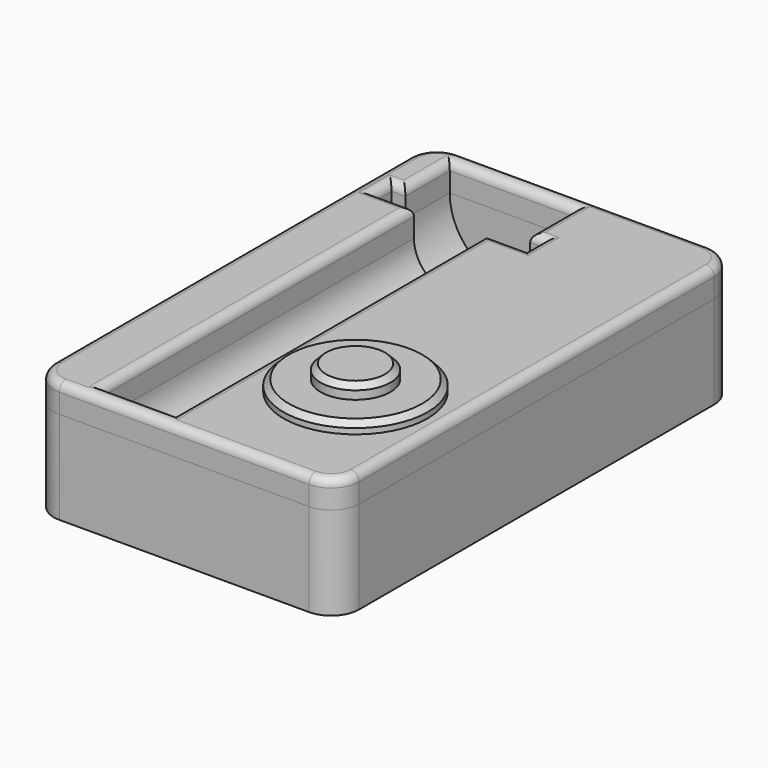
from build123d import *

# Parameters (mm, degrees)
F0_W           = 55
F0_H           = 90
F1_DEPTH       = 16.75
F4_R           = 13
F5_DEPTH       = 2
F7_W           = 55
F7_H           = 90
F8_DEPTH       = 5
F9_R           = 13
F10_DEPTH      = 2
F11_R          = 6.3
F12_DEPTH      = 23.751
F13_R          = 5
F13_2_R        = 5
F14_SIZE       = 1
F15_T1_DEPTH   = 22.5
F15_T3_DEPTH   = 13.75
F15_T5_DEPTH   = 6.25
F15_T7_DEPTH   = 4
F15_T9_DEPTH   = 11
F15_T11_DEPTH  = 73.75
F15_T13_DEPTH  = 13
F15_T15_DEPTH  = 11
F15_T17_DEPTH  = 6.25
F15_T19_DEPTH  = 80
F15_T21_DEPTH  = 45
F15_T24_ANGLE  = 90
F15_T26_ANGLE  = 90
F15_T28_ANGLE  = 90
F15_T30_ANGLE  = 90
F15_T35_DEPTH  = 26.25
F15_T39_DEPTH  = 17.5
F15_T46_DEPTH  = 26.25
F15_T50_DEPTH  = 17.5
F15_T57_DEPTH  = 10
F15_T61_DEPTH  = 7.75
F15_T68_DEPTH  = 7.75
F15_T72_DEPTH  = 14.75
F15_T79_DEPTH  = 77.5
F15_T83_DEPTH  = 16.75
F15_T90_DEPTH  = 77.5
F15_T94_DEPTH  = 16.75
F15_T101_DEPTH = 7.75
F15_T105_DEPTH = 14.75
F15_T112_DEPTH = 10
F15_T116_DEPTH = 7.75
F16_R          = 6.3
F17_DEPTH      = 26.25
F18_SIZE       = 1


# Not quite as in the source:
# - a fillet or chamfer that OpenCascade refuses, or shapes differently, is made with other operations: its cross-section is extruded or revolved along the edge and cut away or added


with BuildPart() as f1:
    # F0 (on Top) → F1 (new body)
    with BuildSketch(Plane.XY):
        Rectangle(F0_W, F0_H)
    extrude(amount=-F1_DEPTH)

    # F2 (on face) → F3 (revolve, cut)
    with BuildSketch(Plane.XY):
        Polygon((0.75, 42), (-10.5, 42), (-10.5, -42), (-4, -42), (-4, 28), (3.25, 28), (3.25, 32), (0.75, 32), align=None)
    revolve(axis=Axis((-10.5, 0, 0), (0, 1, 0)), mode=Mode.SUBTRACT)


with BuildPart() as f5:
    # F4 (on face) → F5 (new body)
    with BuildSketch(Plane.XY):
        with Locations((12.5, -25)):
            Circle(F4_R)
    extrude(amount=F5_DEPTH)


with BuildPart() as f8:
    # F7 (on face) → F8 (new body)
    with BuildSketch(Plane.XY):
        Rectangle(F7_W, F7_H)
        Polygon((-21.75, 42), (0.75, 42), (0.75, 32), (3.25, 32), (3.25, 28), (-4, 28), (-4, -42), (-17, -42), (-17, 28), (-24.25, 28), (-24.25, 32), (-21.75, 32), align=None, mode=Mode.SUBTRACT)
    extrude(amount=F8_DEPTH)


with BuildPart() as f10:
    # F9 (on face) → F10 (new body)
    with BuildSketch(Plane.XY.offset(5)):
        with Locations((11.75, -21.1021695286)):
            Circle(F9_R)
    extrude(amount=F10_DEPTH)


with BuildPart() as f12_tool:
    # F11 (on face) → F12 (new body, through all)
    with BuildSketch(Plane.XY.offset(7)):
        with Locations((11.75, -21.1021695286)):
            Circle(F11_R)
    extrude(amount=-F12_DEPTH)


with BuildPart() as f1_1:
    add(f1.part)

    # F12: cut by f12_tool
    add(f12_tool.part, mode=Mode.SUBTRACT)

    # F13
    f13_edges = [f1_1.edges().sort_by_distance(p)[0] for p in [
        (-27.5, -45, -8.375),
        (27.5, -45, -8.375),
        (27.5, 45, -8.375),
        (-27.5, 45, -8.375),
    ]]
    fillet(f13_edges, radius=F13_R)


with BuildPart() as f8_1:
    add(f8.part)

    # F12: cut by f12_tool
    add(f12_tool.part, mode=Mode.SUBTRACT)

    # F13#2
    f13_2_edges = [f8_1.edges().sort_by_distance(p)[0] for p in [
        (-27.5, -45, 2.5),
        (27.5, -45, 2.5),
        (27.5, 45, 2.5),
        (-27.5, 45, 2.5),
    ]]
    fillet(f13_2_edges, radius=F13_2_R)

    # F15: fillet of radius 1.5 on 13 edges, made by hand

    # F15_s2 → F15_t1 (cut)
    with BuildSketch(Plane.YZ.offset(-21.75)):
        with BuildLine():
            ThreePointArc((43.5, 5), (42.4393398282, 4.5606601718), (42, 3.5))
            Line((42, 3.5), (42, 5))
            Line((42, 5), (43.5, 5))
        make_face()
    extrude(amount=F15_T1_DEPTH, mode=Mode.SUBTRACT)

    # F15_s4 → F15_t3 (cut)
    with BuildSketch(Plane.XZ.offset(-42)):
        with BuildLine():
            ThreePointArc((-23.25, 5), (-22.1893398282, 4.5606601718), (-21.75, 3.5))
            Line((-21.75, 3.5), (-21.75, 5))
            Line((-21.75, 5), (-23.25, 5))
        make_face()
        with BuildLine():
            ThreePointArc((2.25, 5), (1.1893398282, 4.5606601718), (0.75, 3.5))
            Line((0.75, 3.5), (0.75, 5))
            Line((0.75, 5), (2.25, 5))
        make_face()
    extrude(amount=F15_T3_DEPTH, mode=Mode.SUBTRACT)

    # F15_s6 → F15_t5 (cut)
    with BuildSketch(Plane.YZ.offset(-24.25)):
        with BuildLine():
            ThreePointArc((33.5, 5), (32.4393398282, 4.5606601718), (32, 3.5))
            Line((32, 3.5), (32, 5))
            Line((32, 5), (33.5, 5))
        make_face()
    extrude(amount=F15_T5_DEPTH, mode=Mode.SUBTRACT)

    # F15_s8 → F15_t7 (cut)
    with BuildSketch(Plane.XZ.offset(-32)):
        with BuildLine():
            ThreePointArc((-25.75, 5), (-24.6893398282, 4.5606601718), (-24.25, 3.5))
            Line((-24.25, 3.5), (-24.25, 5))
            Line((-24.25, 5), (-25.75, 5))
        make_face()
        with BuildLine():
            ThreePointArc((4.75, 5), (3.6893398282, 4.5606601718), (3.25, 3.5))
            Line((3.25, 3.5), (3.25, 5))
            Line((3.25, 5), (4.75, 5))
        make_face()
    extrude(amount=F15_T7_DEPTH, mode=Mode.SUBTRACT)

    # F15_s10 → F15_t9 (cut)
    with BuildSketch(Plane.YZ.offset(-24.25)):
        with BuildLine():
            ThreePointArc((26.5, 5), (27.5606601718, 4.5606601718), (28, 3.5))
            Line((28, 3.5), (28, 5))
            Line((28, 5), (26.5, 5))
        make_face()
    extrude(amount=F15_T9_DEPTH, mode=Mode.SUBTRACT)

    # F15_s12 → F15_t11 (cut)
    with BuildSketch(Plane.XZ.offset(-31.75)):
        with BuildLine():
            ThreePointArc((-18.5, 5), (-17.4393398282, 4.5606601718), (-17, 3.5))
            Line((-17, 3.5), (-17, 5))
            Line((-17, 5), (-18.5, 5))
        make_face()
        with BuildLine():
            ThreePointArc((-2.5, 5), (-3.5606601718, 4.5606601718), (-4, 3.5))
            Line((-4, 3.5), (-4, 5))
            Line((-4, 5), (-2.5, 5))
        make_face()
    extrude(amount=F15_T11_DEPTH, mode=Mode.SUBTRACT)

    # F15_s14 → F15_t13 (cut)
    with BuildSketch(Plane.YZ.offset(-17)):
        with BuildLine():
            ThreePointArc((-43.5, 5), (-42.4393398282, 4.5606601718), (-42, 3.5))
            Line((-42, 3.5), (-42, 5))
            Line((-42, 5), (-43.5, 5))
        make_face()
    extrude(amount=F15_T13_DEPTH, mode=Mode.SUBTRACT)

    # F15_s16 → F15_t15 (cut)
    with BuildSketch(Plane.YZ.offset(-7.75)):
        with BuildLine():
            ThreePointArc((26.5, 5), (27.5606601718, 4.5606601718), (28, 3.5))
            Line((28, 3.5), (28, 5))
            Line((28, 5), (26.5, 5))
        make_face()
    extrude(amount=F15_T15_DEPTH, mode=Mode.SUBTRACT)

    # F15_s18 → F15_t17 (cut)
    with BuildSketch(Plane.YZ.offset(-3)):
        with BuildLine():
            ThreePointArc((33.5, 5), (32.4393398282, 4.5606601718), (32, 3.5))
            Line((32, 3.5), (32, 5))
            Line((32, 5), (33.5, 5))
        make_face()
    extrude(amount=F15_T17_DEPTH, mode=Mode.SUBTRACT)

    # F15_s20 → F15_t19 (cut)
    with BuildSketch(Plane.XZ.offset(-40)):
        with BuildLine():
            ThreePointArc((26, 5), (27.0606601718, 4.5606601718), (27.5, 3.5))
            Line((27.5, 3.5), (27.5, 5))
            Line((27.5, 5), (26, 5))
        make_face()
        with BuildLine():
            ThreePointArc((-27.5, 3.5), (-27.0606601718, 4.5606601718), (-26, 5))
            Line((-26, 5), (-27.5, 5))
            Line((-27.5, 5), (-27.5, 3.5))
        make_face()
    extrude(amount=F15_T19_DEPTH, mode=Mode.SUBTRACT)

    # F15_s22 → F15_t21 (cut)
    with BuildSketch(Plane.YZ.offset(-22.5)):
        with BuildLine():
            ThreePointArc((43.5, 5), (44.5606601718, 4.5606601718), (45, 3.5))
            Line((45, 3.5), (45, 5))
            Line((45, 5), (43.5, 5))
        make_face()
        with BuildLine():
            ThreePointArc((-43.5, 5), (-44.5606601718, 4.5606601718), (-45, 3.5))
            Line((-45, 3.5), (-45, 5))
            Line((-45, 5), (-43.5, 5))
        make_face()
    extrude(amount=F15_T21_DEPTH, mode=Mode.SUBTRACT)

    # F15_s23 → F15_t24 (revolve, cut)
    with BuildSketch(Plane.YZ.offset(22.5)):
        with BuildLine():
            ThreePointArc((-43.5, 5), (-44.5606601718, 4.5606601718), (-45, 3.5))
            Line((-45, 3.5), (-45, 5))
            Line((-45, 5), (-43.5, 5))
        make_face()
    revolve(axis=Axis((22.5, -40, 5), (0, 0, 1)), revolution_arc=F15_T24_ANGLE, mode=Mode.SUBTRACT)

    # F15_s25 → F15_t26 (revolve, cut)
    with BuildSketch(Plane.YZ.offset(22.5)):
        with BuildLine():
            ThreePointArc((43.5, 5), (44.5606601718, 4.5606601718), (45, 3.5))
            Line((45, 3.5), (45, 5))
            Line((45, 5), (43.5, 5))
        make_face()
    revolve(axis=Axis((22.5, 40, 5), (0, 0, -1)), revolution_arc=F15_T26_ANGLE, mode=Mode.SUBTRACT)

    # F15_s27 → F15_t28 (revolve, cut)
    with BuildSketch(Plane.XZ.offset(-40)):
        with BuildLine():
            ThreePointArc((-27.5, 3.5), (-27.0606601718, 4.5606601718), (-26, 5))
            Line((-26, 5), (-27.5, 5))
            Line((-27.5, 5), (-27.5, 3.5))
        make_face()
    revolve(axis=Axis((-22.5, 40, 5), (0, 0, -1)), revolution_arc=F15_T28_ANGLE, mode=Mode.SUBTRACT)

    # F15_s29 → F15_t30 (revolve, cut)
    with BuildSketch(Plane.XZ.offset(40)):
        with BuildLine():
            ThreePointArc((-27.5, 3.5), (-27.0606601718, 4.5606601718), (-26, 5))
            Line((-26, 5), (-27.5, 5))
            Line((-27.5, 5), (-27.5, 3.5))
        make_face()
    revolve(axis=Axis((-22.5, -40, 5), (0, 0, 1)), revolution_arc=F15_T30_ANGLE, mode=Mode.SUBTRACT)


with BuildPart() as f10_1:
    add(f10.part)

    # F12: cut by f12_tool
    add(f12_tool.part, mode=Mode.SUBTRACT)

    # F14
    f14_edges = [f10_1.edges().sort_by_distance(p)[0] for p in [
        (-1.25, -21.10217, 7),
    ]]
    chamfer(f14_edges, length=F14_SIZE)


with BuildPart() as f15_tool33:
    # F15_s34 → F15_t35 (new body)
    with BuildSketch(Plane.YZ.offset(-25.5)):
        with BuildLine():
            ThreePointArc((43.5, 5), (42.4393398282, 4.5606601718), (42, 3.5))
            Line((42, 3.5), (42, 5))
            Line((42, 5), (43.5, 5))
        make_face()
    extrude(amount=F15_T35_DEPTH)

    split(bisect_by=Plane.YZ.offset(-21.75), keep=Keep.BOTTOM)


with BuildPart() as f15_tool37:
    # F15_s38 → F15_t39 (new body)
    with BuildSketch(Plane.XZ.offset(-28.25)):
        with BuildLine():
            ThreePointArc((-23.25, 5), (-22.1893398282, 4.5606601718), (-21.75, 3.5))
            Line((-21.75, 3.5), (-21.75, 5))
            Line((-21.75, 5), (-23.25, 5))
        make_face()
    extrude(amount=-F15_T39_DEPTH)

    split(bisect_by=Plane.XZ.offset(-42), keep=Keep.BOTTOM)


with BuildPart() as f15_tool33_1:
    add(f15_tool33.part)

    # F15_t41: intersect F15_tool37
    add(f15_tool37.part, mode=Mode.INTERSECT)


with BuildPart() as f8_2:
    add(f8_1.part)

    # F15_t31: cut F15_tool33
    add(f15_tool33_1.part, mode=Mode.SUBTRACT)


with BuildPart() as f15_tool44:
    # F15_s45 → F15_t46 (new body)
    with BuildSketch(Plane.YZ.offset(-21.75)):
        with BuildLine():
            ThreePointArc((43.5, 5), (42.4393398282, 4.5606601718), (42, 3.5))
            Line((42, 3.5), (42, 5))
            Line((42, 5), (43.5, 5))
        make_face()
    extrude(amount=F15_T46_DEPTH)

    split(bisect_by=Plane.YZ.offset(0.75), keep=Keep.TOP)


with BuildPart() as f15_tool48:
    # F15_s49 → F15_t50 (new body)
    with BuildSketch(Plane.XZ.offset(-45.75)):
        with BuildLine():
            ThreePointArc((2.25, 5), (1.1893398282, 4.5606601718), (0.75, 3.5))
            Line((0.75, 3.5), (0.75, 5))
            Line((0.75, 5), (2.25, 5))
        make_face()
    extrude(amount=F15_T50_DEPTH)

    split(bisect_by=Plane.XZ.offset(-42), keep=Keep.BOTTOM)


with BuildPart() as f15_tool44_1:
    add(f15_tool44.part)

    # F15_t52: intersect F15_tool48
    add(f15_tool48.part, mode=Mode.INTERSECT)


with BuildPart() as f8_3:
    add(f8_2.part)

    # F15_t42: cut F15_tool44
    add(f15_tool44_1.part, mode=Mode.SUBTRACT)


with BuildPart() as f15_tool55:
    # F15_s56 → F15_t57 (new body)
    with BuildSketch(Plane.YZ.offset(-28)):
        with BuildLine():
            ThreePointArc((33.5, 5), (32.4393398282, 4.5606601718), (32, 3.5))
            Line((32, 3.5), (32, 5))
            Line((32, 5), (33.5, 5))
        make_face()
    extrude(amount=F15_T57_DEPTH)

    split(bisect_by=Plane.YZ.offset(-24.25), keep=Keep.BOTTOM)


with BuildPart() as f15_tool59:
    # F15_s60 → F15_t61 (new body)
    with BuildSketch(Plane.XZ.offset(-28)):
        with BuildLine():
            ThreePointArc((-25.75, 5), (-24.6893398282, 4.5606601718), (-24.25, 3.5))
            Line((-24.25, 3.5), (-24.25, 5))
            Line((-24.25, 5), (-25.75, 5))
        make_face()
    extrude(amount=-F15_T61_DEPTH)

    split(bisect_by=Plane.XZ.offset(-32), keep=Keep.BOTTOM)


with BuildPart() as f15_tool55_1:
    add(f15_tool55.part)

    # F15_t63: intersect F15_tool59
    add(f15_tool59.part, mode=Mode.INTERSECT)


with BuildPart() as f8_4:
    add(f8_3.part)

    # F15_t53: cut F15_tool55
    add(f15_tool55_1.part, mode=Mode.SUBTRACT)


with BuildPart() as f15_tool66:
    # F15_s67 → F15_t68 (new body)
    with BuildSketch(Plane.XZ.offset(-24.25)):
        with BuildLine():
            ThreePointArc((-25.75, 5), (-24.6893398282, 4.5606601718), (-24.25, 3.5))
            Line((-24.25, 3.5), (-24.25, 5))
            Line((-24.25, 5), (-25.75, 5))
        make_face()
    extrude(amount=-F15_T68_DEPTH)

    split(bisect_by=Plane.XZ.offset(-28), keep=Keep.TOP)


with BuildPart() as f15_tool70:
    # F15_s71 → F15_t72 (new body)
    with BuildSketch(Plane.YZ.offset(-13.25)):
        with BuildLine():
            ThreePointArc((26.5, 5), (27.5606601718, 4.5606601718), (28, 3.5))
            Line((28, 3.5), (28, 5))
            Line((28, 5), (26.5, 5))
        make_face()
    extrude(amount=-F15_T72_DEPTH)

    split(bisect_by=Plane.YZ.offset(-24.25), keep=Keep.BOTTOM)


with BuildPart() as f15_tool66_1:
    add(f15_tool66.part)

    # F15_t74: intersect F15_tool70
    add(f15_tool70.part, mode=Mode.INTERSECT)


with BuildPart() as f8_5:
    add(f8_4.part)

    # F15_t64: cut F15_tool66
    add(f15_tool66_1.part, mode=Mode.SUBTRACT)


with BuildPart() as f15_tool77:
    # F15_s78 → F15_t79 (new body)
    with BuildSketch(Plane.XZ.offset(45.75)):
        with BuildLine():
            ThreePointArc((-18.5, 5), (-17.4393398282, 4.5606601718), (-17, 3.5))
            Line((-17, 3.5), (-17, 5))
            Line((-17, 5), (-18.5, 5))
        make_face()
    extrude(amount=-F15_T79_DEPTH)

    split(bisect_by=Plane.XZ.offset(42), keep=Keep.TOP)


with BuildPart() as f15_tool81:
    # F15_s82 → F15_t83 (new body)
    with BuildSketch(Plane.YZ.offset(-4)):
        with BuildLine():
            ThreePointArc((-43.5, 5), (-42.4393398282, 4.5606601718), (-42, 3.5))
            Line((-42, 3.5), (-42, 5))
            Line((-42, 5), (-43.5, 5))
        make_face()
    extrude(amount=-F15_T83_DEPTH)

    split(bisect_by=Plane.YZ.offset(-17), keep=Keep.BOTTOM)


with BuildPart() as f15_tool77_1:
    add(f15_tool77.part)

    # F15_t85: intersect F15_tool81
    add(f15_tool81.part, mode=Mode.INTERSECT)


with BuildPart() as f8_6:
    add(f8_5.part)

    # F15_t75: cut F15_tool77
    add(f15_tool77_1.part, mode=Mode.SUBTRACT)


with BuildPart() as f15_tool88:
    # F15_s89 → F15_t90 (new body)
    with BuildSketch(Plane.XZ.offset(-31.75)):
        with BuildLine():
            ThreePointArc((-2.5, 5), (-3.5606601718, 4.5606601718), (-4, 3.5))
            Line((-4, 3.5), (-4, 5))
            Line((-4, 5), (-2.5, 5))
        make_face()
    extrude(amount=F15_T90_DEPTH)

    split(bisect_by=Plane.XZ.offset(42), keep=Keep.TOP)


with BuildPart() as f15_tool92:
    # F15_s93 → F15_t94 (new body)
    with BuildSketch(Plane.YZ.offset(-0.25)):
        with BuildLine():
            ThreePointArc((-43.5, 5), (-42.4393398282, 4.5606601718), (-42, 3.5))
            Line((-42, 3.5), (-42, 5))
            Line((-42, 5), (-43.5, 5))
        make_face()
    extrude(amount=-F15_T94_DEPTH)

    split(bisect_by=Plane.YZ.offset(-4), keep=Keep.TOP)


with BuildPart() as f15_tool88_1:
    add(f15_tool88.part)

    # F15_t96: intersect F15_tool92
    add(f15_tool92.part, mode=Mode.INTERSECT)


with BuildPart() as f8_7:
    add(f8_6.part)

    # F15_t86: cut F15_tool88
    add(f15_tool88_1.part, mode=Mode.SUBTRACT)


with BuildPart() as f15_tool99:
    # F15_s100 → F15_t101 (new body)
    with BuildSketch(Plane.XZ.offset(-32)):
        with BuildLine():
            ThreePointArc((4.75, 5), (3.6893398282, 4.5606601718), (3.25, 3.5))
            Line((3.25, 3.5), (3.25, 5))
            Line((3.25, 5), (4.75, 5))
        make_face()
    extrude(amount=F15_T101_DEPTH)

    split(bisect_by=Plane.XZ.offset(-28), keep=Keep.TOP)


with BuildPart() as f15_tool103:
    # F15_s104 → F15_t105 (new body)
    with BuildSketch(Plane.YZ.offset(7)):
        with BuildLine():
            ThreePointArc((26.5, 5), (27.5606601718, 4.5606601718), (28, 3.5))
            Line((28, 3.5), (28, 5))
            Line((28, 5), (26.5, 5))
        make_face()
    extrude(amount=-F15_T105_DEPTH)

    split(bisect_by=Plane.YZ.offset(3.25), keep=Keep.TOP)


with BuildPart() as f15_tool99_1:
    add(f15_tool99.part)

    # F15_t107: intersect F15_tool103
    add(f15_tool103.part, mode=Mode.INTERSECT)


with BuildPart() as f8_8:
    add(f8_7.part)

    # F15_t97: cut F15_tool99
    add(f15_tool99_1.part, mode=Mode.SUBTRACT)


with BuildPart() as f15_tool110:
    # F15_s111 → F15_t112 (new body)
    with BuildSketch(Plane.YZ.offset(-3)):
        with BuildLine():
            ThreePointArc((33.5, 5), (32.4393398282, 4.5606601718), (32, 3.5))
            Line((32, 3.5), (32, 5))
            Line((32, 5), (33.5, 5))
        make_face()
    extrude(amount=F15_T112_DEPTH)

    split(bisect_by=Plane.YZ.offset(3.25), keep=Keep.TOP)


with BuildPart() as f15_tool114:
    # F15_s115 → F15_t116 (new body)
    with BuildSketch(Plane.XZ.offset(-35.75)):
        with BuildLine():
            ThreePointArc((4.75, 5), (3.6893398282, 4.5606601718), (3.25, 3.5))
            Line((3.25, 3.5), (3.25, 5))
            Line((3.25, 5), (4.75, 5))
        make_face()
    extrude(amount=F15_T116_DEPTH)

    split(bisect_by=Plane.XZ.offset(-32), keep=Keep.BOTTOM)


with BuildPart() as f15_tool110_1:
    add(f15_tool110.part)

    # F15_t118: intersect F15_tool114
    add(f15_tool114.part, mode=Mode.INTERSECT)


with BuildPart() as f8_9:
    add(f8_8.part)

    # F15_t108: cut F15_tool110
    add(f15_tool110_1.part, mode=Mode.SUBTRACT)


with BuildPart() as f17:
    # F16 (on face) → F17 (new body)
    with BuildSketch(Plane(origin=(0, 0, -16.75), x_dir=(1, 0, 0), z_dir=(0, 0, -1))):
        with Locations((11.75, 21.1021695286)):
            Circle(F16_R)
    extrude(amount=-F17_DEPTH)

    # F18
    f18_edges = [f17.edges().sort_by_distance(p)[0] for p in [
        (5.45, -21.10217, 9.5),
    ]]
    chamfer(f18_edges, length=F18_SIZE)


solid = Compound([f1_1.part, f10_1.part, f8_9.part, f17.part])
